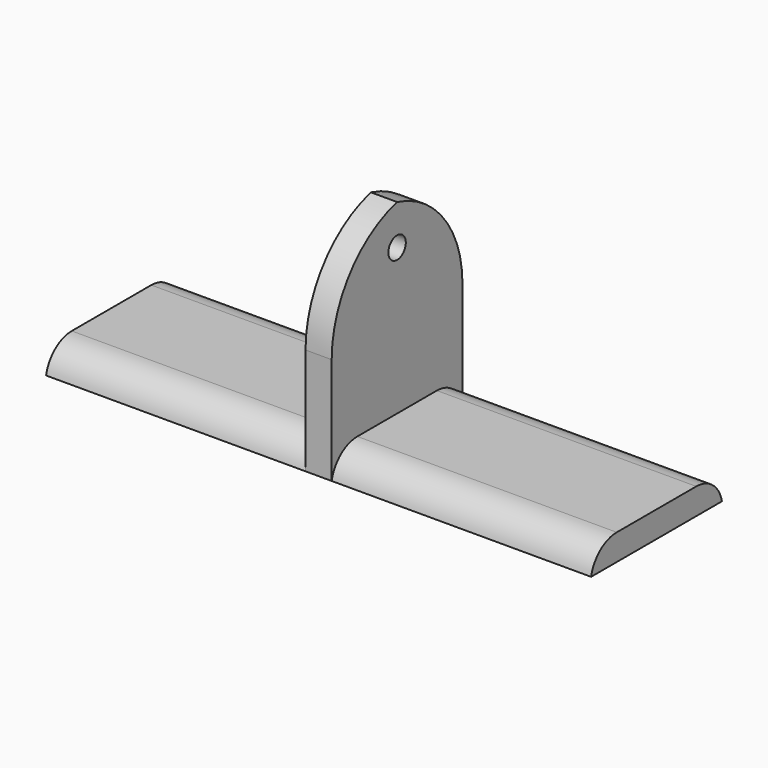
from build123d import *

# Parameters (mm, degrees)
F0_W         = 50
F0_H         = 15
F2_DEPTH     = 2.4
F3_W         = 2.4
F3_H         = 15
F4_DEPTH     = 17.4
F6_T1_DEPTH  = 52.4
F5_R         = 1
F7_DEPTH     = 26.201
F8_T1_DEPTH  = 31.1484692284
F8_T3_DEPTH  = 31.1484692284
F8_T8_DEPTH  = 38.4969384567
F8_T13_DEPTH = 38.4969384567
F8_T18_DEPTH = 38.4969384567
F8_T23_DEPTH = 38.4969384567


# Not quite as in the source:
# - a fillet or chamfer that OpenCascade refuses, or shapes differently, is made with other operations: its cross-section is extruded or revolved along the edge and cut away or added


with BuildPart() as f2:
    # F0 (on Top) → F2 (new body)
    with BuildSketch(Plane.XY):
        Rectangle(F0_W, F0_H)
    extrude(amount=F2_DEPTH)

    # F3 (on face) → F4 (join)
    with BuildSketch(Plane.XY.offset(2.4)):
        Rectangle(F3_W, F3_H)
    extrude(amount=F4_DEPTH)

    # F6: fillet of radius 10 on 2 edges, made by hand

    # F6_s2 → F6_t1 (cut)
    with BuildSketch(Plane.YZ.offset(-26.2)):
        with BuildLine():
            ThreePointArc((-7.5, 9.8), (-4.5710678119, 16.8710678119), (2.5, 19.8))
            Line((2.5, 19.8), (-7.5, 19.8))
            Line((-7.5, 19.8), (-7.5, 9.8))
        make_face()
        with BuildLine():
            ThreePointArc((7.5, 9.8), (4.5710678119, 16.8710678119), (-2.5, 19.8))
            Line((-2.5, 19.8), (7.5, 19.8))
            Line((7.5, 19.8), (7.5, 9.8))
        make_face()
    extrude(amount=F6_T1_DEPTH, mode=Mode.SUBTRACT)

    # F5 (on face) → F7 (cut, through all)
    with BuildSketch(Plane.YZ.offset(1.2)):
        with Locations((0, 15.8)):
            Circle(F5_R)
    extrude(amount=-F7_DEPTH, mode=Mode.SUBTRACT)

    # F8: fillet of radius 3 on 4 edges, made by hand

    # F8_s2 → F8_t1 (cut)
    with BuildSketch(Plane.YZ.offset(-32.3484692284)):
        with BuildLine():
            ThreePointArc((-4.5606123087, 2.4), (-6.4579789048, 1.7237900077), (-7.5, 0))
            Line((-7.5, 0), (-7.5, 2.4))
            Line((-7.5, 2.4), (-4.5606123087, 2.4))
        make_face()
        with BuildLine():
            ThreePointArc((7.5, 0), (6.4579789048, 1.7237900077), (4.5606123087, 2.4))
            Line((4.5606123087, 2.4), (7.5, 2.4))
            Line((7.5, 2.4), (7.5, 0))
        make_face()
    extrude(amount=F8_T1_DEPTH, mode=Mode.SUBTRACT)

    # F8_s4 → F8_t3 (cut)
    with BuildSketch(Plane.YZ.offset(1.2)):
        with BuildLine():
            ThreePointArc((-4.5606123087, 2.4), (-6.4579789048, 1.7237900077), (-7.5, 0))
            Line((-7.5, 0), (-7.5, 2.4))
            Line((-7.5, 2.4), (-4.5606123087, 2.4))
        make_face()
        with BuildLine():
            ThreePointArc((7.5, 0), (6.4579789048, 1.7237900077), (4.5606123087, 2.4))
            Line((4.5606123087, 2.4), (7.5, 2.4))
            Line((7.5, 2.4), (7.5, 0))
        make_face()
    extrude(amount=F8_T3_DEPTH, mode=Mode.SUBTRACT)


with BuildPart() as f8_tool6:
    # F8_s7 → F8_t8 (new body)
    with BuildSketch(Plane.YZ.offset(-32.3484692284)):
        with BuildLine():
            ThreePointArc((-4.5606123087, 2.4), (-6.4579789048, 1.7237900077), (-7.5, 0))
            Line((-7.5, 0), (-7.5, 2.4))
            Line((-7.5, 2.4), (-4.5606123087, 2.4))
        make_face()
    extrude(amount=F8_T8_DEPTH)

    split(bisect_by=Plane.YZ.offset(1.2), keep=Keep.TOP)


with BuildPart() as f2_1:
    add(f2.part)

    # F8_t5: cut F8_tool6
    add(f8_tool6.part, mode=Mode.SUBTRACT)


with BuildPart() as f8_tool11:
    # F8_s12 → F8_t13 (new body)
    with BuildSketch(Plane.YZ.offset(-6.1484692284)):
        with BuildLine():
            ThreePointArc((-4.5606123087, 2.4), (-6.4579789048, 1.7237900077), (-7.5, 0))
            Line((-7.5, 0), (-7.5, 2.4))
            Line((-7.5, 2.4), (-4.5606123087, 2.4))
        make_face()
    extrude(amount=F8_T13_DEPTH)

    split(bisect_by=Plane.YZ.offset(-1.2), keep=Keep.BOTTOM)


with BuildPart() as f2_2:
    add(f2_1.part)

    # F8_t10: cut F8_tool11
    add(f8_tool11.part, mode=Mode.SUBTRACT)


with BuildPart() as f8_tool16:
    # F8_s17 → F8_t18 (new body)
    with BuildSketch(Plane.YZ.offset(32.3484692284)):
        with BuildLine():
            ThreePointArc((7.5, 0), (6.4579789048, 1.7237900077), (4.5606123087, 2.4))
            Line((4.5606123087, 2.4), (7.5, 2.4))
            Line((7.5, 2.4), (7.5, 0))
        make_face()
    extrude(amount=-F8_T18_DEPTH)

    split(bisect_by=Plane.YZ.offset(-1.2), keep=Keep.BOTTOM)


with BuildPart() as f2_3:
    add(f2_2.part)

    # F8_t15: cut F8_tool16
    add(f8_tool16.part, mode=Mode.SUBTRACT)


with BuildPart() as f8_tool21:
    # F8_s22 → F8_t23 (new body)
    with BuildSketch(Plane.YZ.offset(6.1484692284)):
        with BuildLine():
            ThreePointArc((7.5, 0), (6.4579789048, 1.7237900077), (4.5606123087, 2.4))
            Line((4.5606123087, 2.4), (7.5, 2.4))
            Line((7.5, 2.4), (7.5, 0))
        make_face()
    extrude(amount=-F8_T23_DEPTH)

    split(bisect_by=Plane.YZ.offset(1.2), keep=Keep.TOP)


with BuildPart() as f2_4:
    add(f2_3.part)

    # F8_t20: cut F8_tool21
    add(f8_tool21.part, mode=Mode.SUBTRACT)


solid = f2_4.part
